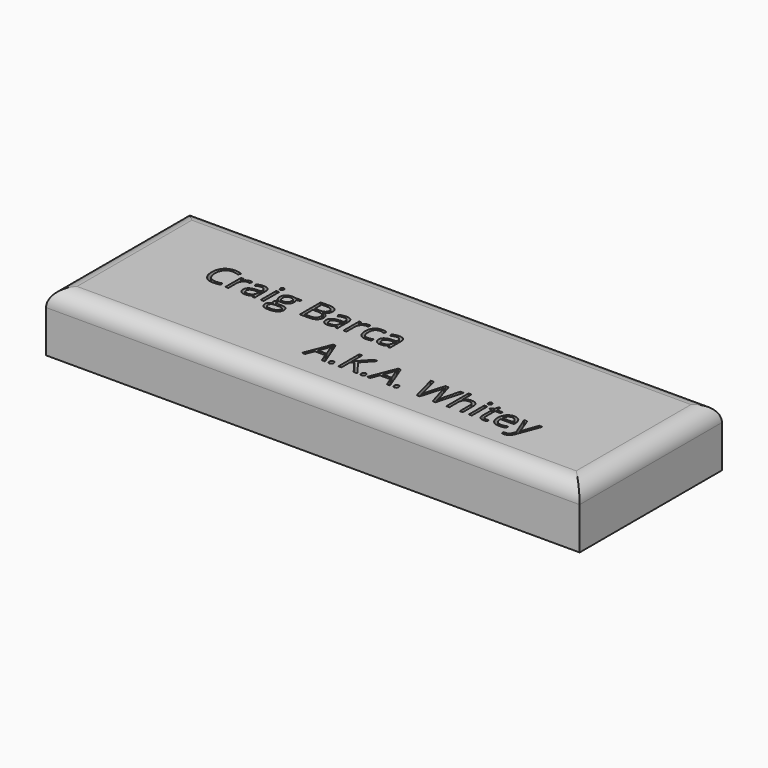
from build123d import *

# Parameters (mm, degrees)
F0_W         = 57.15
F0_H         = 19.05
F1_DEPTH     = 6.35
F2_R         = 1.8396307345
F3_TEXT_SIZE = 3.9173142705
F4_DEPTH     = 3.175


# Not quite as in the source:
# - Text() gives the source's letters only with a copy of the font that has no kerning and outlines rounded to 1/6400 em; it was checked with that copy


with BuildPart() as f1:
    # F0 (on Top) → F1 (new body)
    with BuildSketch(Plane.XY):
        Rectangle(F0_W, F0_H)
    extrude(amount=F1_DEPTH)

    # F2
    f2_edges = [f1.edges().sort_by_distance(p)[0] for p in [
        (0, 9.525, 6.35),
        (-28.575, 0, 6.35),
        (0, -9.525, 6.35),
        (28.575, 0, 6.35),
    ]]
    fillet(f2_edges, radius=F2_R)

    # F3 (on face) → F4 (cut)
    with BuildSketch(Plane.XY.offset(6.35)):
        with Locations((-19.8011055166, 0)):
            Text('Craig Barca', F3_TEXT_SIZE, font='Open Sans', text_align=(TextAlign.LEFT, TextAlign.BOTTOM))
        with Locations((-4.5327610672, -5.3275474078)):
            Text('A.K.A. Whitey', F3_TEXT_SIZE, font='Open Sans', text_align=(TextAlign.LEFT, TextAlign.BOTTOM))
    extrude(amount=-F4_DEPTH, mode=Mode.SUBTRACT)


solid = f1.part
